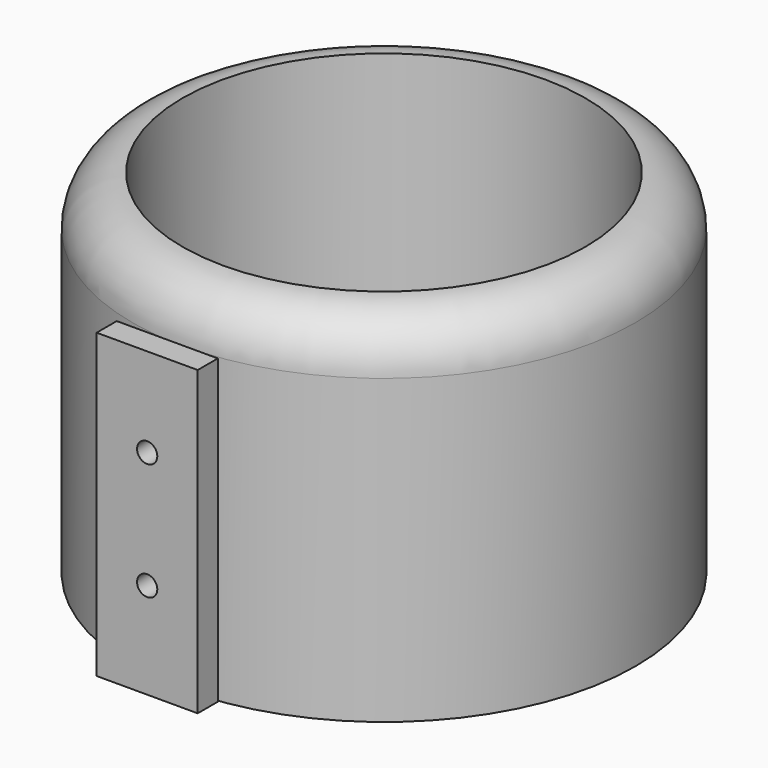
from build123d import *

# Parameters (mm, degrees)
F2_DEPTH   = 76.2
F4_W       = 25.5275620148
F4_H       = 76.3463266194
F5_DEPTH   = 6.35
F9_D       = 5.1054
F9_DEPTH   = 38.1
F9_TIP     = 1.5338169022
F9_2_D     = 5.1054
F9_2_DEPTH = 38.1
F9_2_TIP   = 1.5338169022
F12_DEPTH  = 6.35


# Not quite as in the source:
# - a feature of the source that left no trace in its solid (it failed there, or was rolled back) is left out


with BuildPart() as f1:
    # F0 (on Front) → F1 (revolve)
    with BuildSketch(Plane.XZ):
        with BuildLine():
            Line((54.6532709479, 45.5005168915), (3.770736279, 45.5005168915))
            Line((3.770736279, 45.5005168915), (3.770736279, -43.609585613))
            Line((3.770736279, -43.609585613), (67.3532709479, -43.609585613))
            Line((67.3532709479, -43.609585613), (67.3532709479, 32.8005168915))
            ThreePointArc((67.3532709479, 32.8005168915), (63.633527069, 41.7807730125), (54.6532709479, 45.5005168915))
        make_face()
    revolve(axis=Axis((3.770736279, 0, 0.9454656392), (0, 0, 1)))

    # F2 (cut): a face of the model
    f2_faces = [f1.faces().sort_by_distance(p)[0] for p in [
        (3.770736279, 0, 45.5005168915),
    ]]
    extrude(f2_faces, amount=-F2_DEPTH, mode=Mode.SUBTRACT)

    # F9
    with Locations(Plane.XZ.offset(70.0532)):
        with Locations((0, 10.4649914429), (0, -19.1282723099)):
            Hole(F9_D / 2, depth=F9_DEPTH)
            with Locations((0, 0, -(F9_DEPTH + F9_TIP / 2))):  # 118° drill point
                Cone(0, F9_D / 2, F9_TIP, mode=Mode.SUBTRACT)

    # F11 (on offset) → F12 (cut)
    with BuildSketch(Plane.XY.offset(-25.4)):
        with BuildLine():
            Line((-14.1898515568, -3.9695769455), (3.7818609271, -29.1912425309))
            Line((3.7818609271, -29.1912425309), (24.7812050342, -4.254519477))
            ThreePointArc((24.7812050342, -4.254519477), (27.4402781426, 0.33711338), (28.3639580011, 5.5621088449))
            Line((28.3639580011, 5.5621088449), (28.3639580011, 16.6845112958))
            ThreePointArc((28.3639580011, 16.6845112958), (25.3632832083, 24.8828703101), (17.7792193355, 29.2071176335))
            ThreePointArc((17.7792193355, 29.2071176335), (14.0594292862, 27.6952065298), (11.2158715142, 24.860265191))
            Line((11.2158715142, 24.860265191), (6.6803421116, 18.0569709152))
            Line((6.6803421116, 18.0569709152), (2.9480526056, 24.3856378285))
            ThreePointArc((2.9480526056, 24.3856378285), (-0.4625819691, 27.8674846274), (-5.1023244743, 29.3602923235))
            ThreePointArc((-5.1023244743, 29.3602923235), (-13.5716495731, 25.3831851413), (-17.0183759183, 16.6845112958))
            Line((-17.0183759183, 16.6845112958), (-17.0183759183, 4.8742272403))
            ThreePointArc((-17.0183759183, 4.8742272403), (-16.2940310659, 0.2316680716), (-14.1898515568, -3.9695769455))
        make_face()
    extrude(amount=-F12_DEPTH, mode=Mode.SUBTRACT)


with BuildPart() as f5:
    # F4 (on offset) → F5 (new body)
    with BuildSketch(Plane.XZ.offset(63.7032)):
        with Locations((-4.657e-07, -5.2000600845)):
            Rectangle(F4_W, F4_H)
    extrude(amount=F5_DEPTH)

    # F9#2
    with Locations(Plane.XZ.offset(70.0532)):
        with Locations((0, 10.4649914429), (0, -19.1282723099)):
            Hole(F9_2_D / 2, depth=F9_2_DEPTH)
            with Locations((0, 0, -(F9_2_DEPTH + F9_2_TIP / 2))):  # 118° drill point
                Cone(0, F9_2_D / 2, F9_2_TIP, mode=Mode.SUBTRACT)


solid = Compound([f1.part, f5.part])
